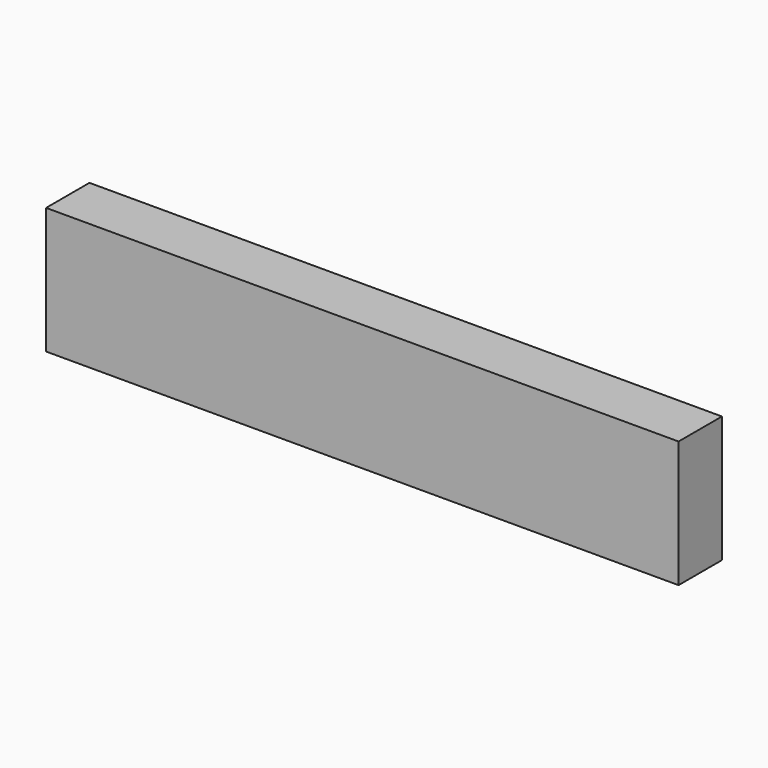
from build123d import *

# Parameters (mm, degrees)
F0_W     = 38.1
F0_H     = 88.9
F1_DEPTH = 222.25


with BuildPart() as f1:
    # F0 (on Right) → F1 (new body, symmetric)
    with BuildSketch(Plane.YZ):
        Rectangle(F0_W, F0_H)
    extrude(amount=F1_DEPTH, both=True)


solid = f1.part
